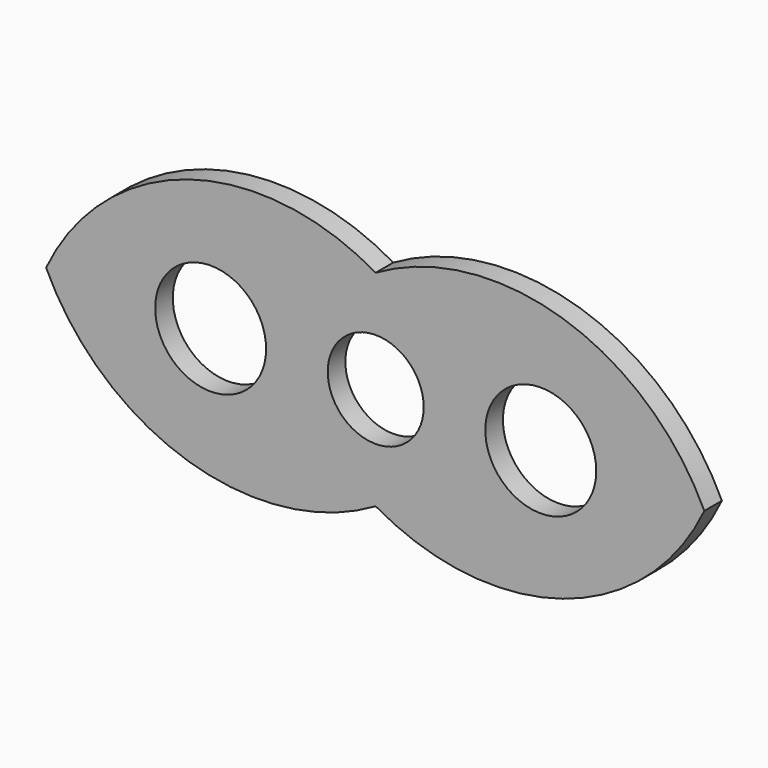
from build123d import *

# Parameters (mm, degrees)
F0_R     = 12.6
F0_R_2   = 10.9
F1_DEPTH = 5


# Not quite as in the source:
# - a feature names something its author has since deleted; it is built from what else it names


with BuildPart() as f1:
    # F0 (on Front) → F1 (new body)
    with BuildSketch(Plane.XZ):
        with BuildLine():
            ThreePointArc((74.653416872, 0), (42.4496947935, 28.0524969579), (0, 23.3572106808))
            ThreePointArc((0, 23.3572106808), (-42.5884817576, 28.1732918571), (-74.8876929283, 0))
            ThreePointArc((-74.8876929283, 0), (-42.5885090722, -28.1733794331), (0, -23.3572106808))
            ThreePointArc((0, -23.3572106808), (42.4496947935, -28.0524969579), (74.653416872, 0))
        make_face()
        with Locations((-37.5000350177, 0)):
            Circle(F0_R, mode=Mode.SUBTRACT)
        Circle(F0_R_2, mode=Mode.SUBTRACT)
        with Locations((37.5000350177, 0)):
            Circle(F0_R, mode=Mode.SUBTRACT)
    extrude(amount=F1_DEPTH)


solid = f1.part
